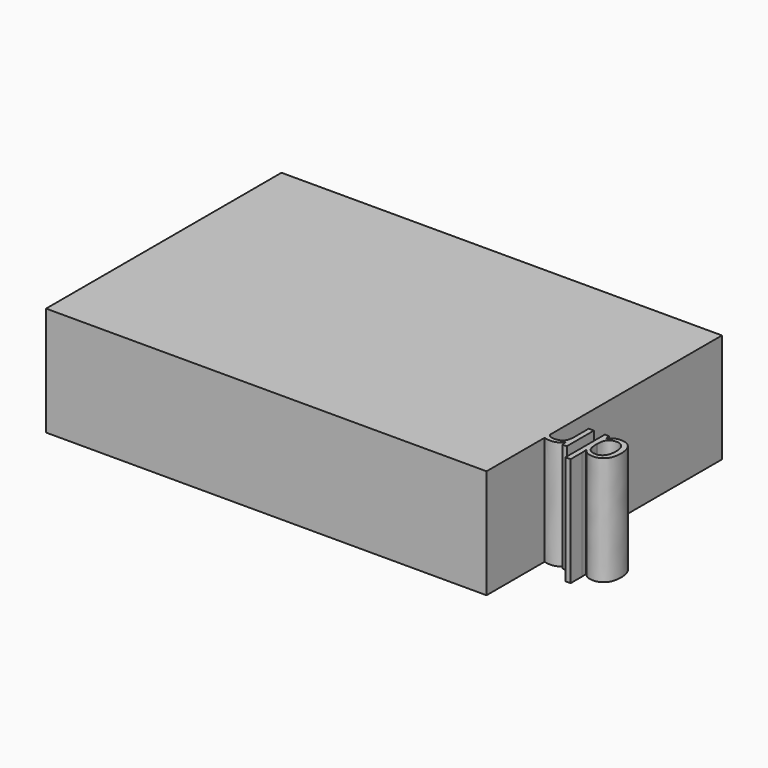
from build123d import *

# Parameters (mm, degrees)
F0_W         = 102.4838387966
F0_H         = 68.4608519077
F1_DEPTH     = 25.4
F2_TEXT_SIZE = 14.7558245083
F3_DEPTH     = 25.4


# Not quite as in the source:
# - Text() gives the source's letters only with a copy of the font that has no kerning and outlines rounded to 1/6400 em; it was checked with that copy


with BuildPart() as f1:
    # F0 (on Top) → F1 (new body)
    with BuildSketch(Plane.XY):
        with Locations((-3.3193379641, 17.4264162779)):
            Rectangle(F0_W, F0_H)
    extrude(amount=F1_DEPTH)

    # F2 (on face) → F3 (join)
    with BuildSketch(Plane.XY.offset(25.4)):
        with Locations((-12.6063059477, 0)):
            Text('yo what up', F2_TEXT_SIZE, font='Open Sans', text_align=(TextAlign.LEFT, TextAlign.BOTTOM))
    extrude(amount=-F3_DEPTH)


solid = f1.part
